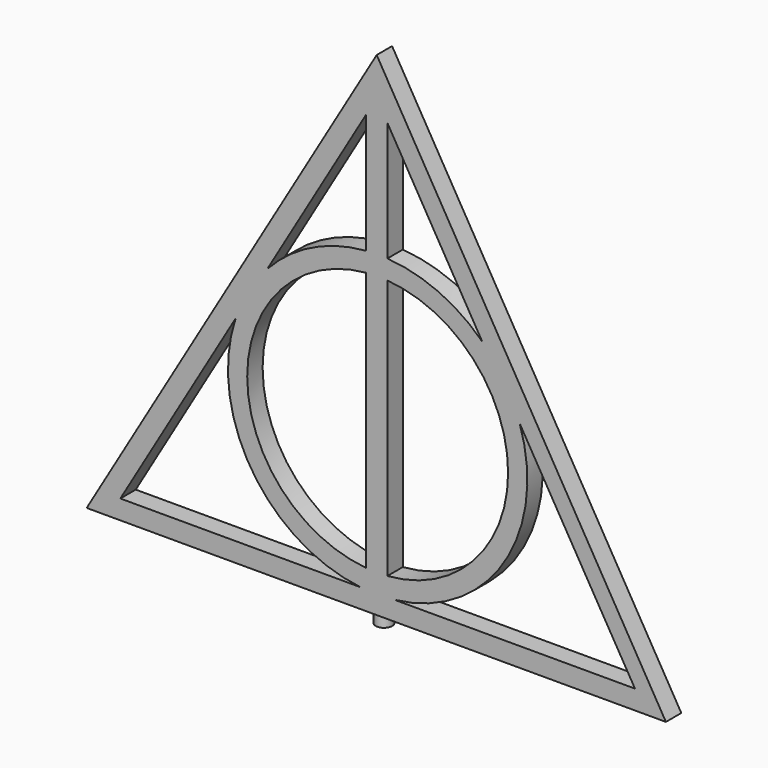
from build123d import *

# Parameters (mm, degrees)
F1_DEPTH = 3.5
F2_R     = 1.5
F3_DEPTH = 2


# Not quite as in the source:
# - a feature names something its author has since deleted; it is built from what else it names


with BuildPart() as f1:
    # F0 (on Front) → F1 (new body)
    with BuildSketch(Plane.XZ):
        Polygon((42.7356177972, 8.1960540903), (-9.8386000647, 97.8239037067), (-62.5526416078, 8.1960540903), align=None)
        with BuildLine():
            Line((-12.7572676559, 11.6960540903), (-56.4336672666, 11.6960540903))
            Line((-56.4336672666, 11.6960540903), (-35.4842691453, 47.3155863706))
            ThreePointArc((-35.4842691453, 47.3155863706), (-32.6024132797, 24.0941164977), (-12.7572676559, 11.6960540903))
        make_face(mode=Mode.SUBTRACT)
        with BuildLine():
            ThreePointArc((-11.7914030425, 15.1152742164), (-33.3740588193, 38.7305133045), (-11.7914030425, 62.3457523925))
            Line((-11.7914030425, 62.3457523925), (-11.7914030425, 15.1152742164))
        make_face(mode=Mode.SUBTRACT)
        with BuildLine():
            ThreePointArc((-6.5689498166, 11.6960540903), (13.2761958072, 24.0941164977), (16.1580516728, 47.3155863706))
            Line((16.1580516728, 47.3155863706), (37.1074497941, 11.6960540903))
            Line((37.1074497941, 11.6960540903), (-6.5689498166, 11.6960540903))
        make_face(mode=Mode.SUBTRACT)
        with BuildLine():
            ThreePointArc((-7.8989818992, 62.3757456007), (14.0478413468, 38.7305133045), (-7.8989818992, 15.0852810082))
            Line((-7.8989818992, 15.0852810082), (-7.8989818992, 62.3757456007))
        make_face(mode=Mode.SUBTRACT)
        with BuildLine():
            Line((-29.7147789735, 57.1252496473), (-11.7914030425, 87.5997417472))
            Line((-11.7914030425, 87.5997417472), (-11.7914030425, 65.8581038309))
            ThreePointArc((-11.7914030425, 65.8581038309), (-21.5817241061, 63.1923695727), (-29.7147789735, 57.1252496473))
        make_face(mode=Mode.SUBTRACT)
        with BuildLine():
            Line((-7.8989818992, 65.8842176728), (-7.8989818992, 87.5997417472))
            Line((-7.8989818992, 87.5997417472), (9.3459755849, 58.2007602904))
            ThreePointArc((9.3459755849, 58.2007602904), (1.4112063573, 63.5860026304), (-7.8989818992, 65.8842176728))
        make_face(mode=Mode.SUBTRACT)
    extrude(amount=F1_DEPTH)

    # F2 (on face) → F3 (join)
    with BuildSketch(Plane(origin=(0, 0, 8.1960540903), x_dir=(1, 0, 0), z_dir=(0, 0, -1))):
        with Locations((-9.9085119053, 1.75)):
            Circle(F2_R)
    extrude(amount=F3_DEPTH)


solid = f1.part
